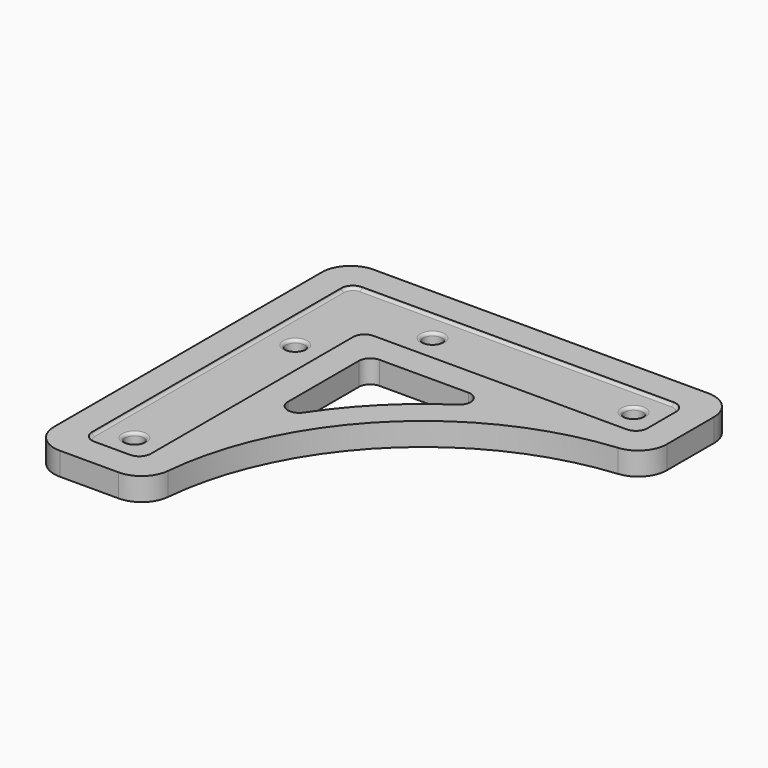
from build123d import *

# Parameters (mm, degrees)
F1_DEPTH = 4
F2_R     = 1.6
F3_DEPTH = 4.001
F4_R     = 5
F5_R     = 1.6
F6_DEPTH = 0.5
F7_R     = 0.49999
F9_DEPTH = 4.001
F10_R    = 2


# Not quite as in the source:
# - a fillet or chamfer is up to 0.001 mm smaller than in the source, because OpenCascade refuses the exact size


with BuildPart() as f1:
    # F0 (on Top) → F1 (new body)
    with BuildSketch(Plane.XY):
        with BuildLine():
            Line((34.1421356237, 14.1421356237), (34.1421356237, 34.1421356237))
            Line((34.1421356237, 34.1421356237), (-34.1421356237, 34.1421356237))
            Line((-34.1421356237, 34.1421356237), (-34.1421356237, -34.1421356237))
            Line((-34.1421356237, -34.1421356237), (-14.1421356237, -34.1421356237))
            ThreePointArc((-14.1421356237, -34.1421356237), (0, 0), (34.1421356237, 14.1421356237))
        make_face()
    extrude(amount=F1_DEPTH)

    # F2 (on face) → F3 (cut, through all)
    with BuildSketch(Plane.XY.offset(4)):
        with Locations((-24.1421356237, -24.1421356237)):
            Circle(F2_R)
        with Locations((-10.8578643763, 24.1421356237)):
            Circle(F2_R)
        with Locations((24.1421356237, 24.1421356237)):
            Circle(F2_R)
        with Locations((-24.1421356237, 10.8578643763)):
            Circle(F2_R)
    extrude(amount=-F3_DEPTH, mode=Mode.SUBTRACT)

    # F4
    f4_edges = [f1.edges().sort_by_distance(p)[0] for p in [
        (-14.142136, -34.142136, 2),
        (-34.142136, -34.142136, 2),
        (34.142136, 14.142136, 2),
        (34.142136, 34.142136, 2),
        (-34.142136, 34.142136, 2),
    ]]
    fillet(f4_edges, radius=F4_R)

    # F5 (on face) → F6 (cut)
    with BuildSketch(Plane.XY.offset(4)):
        with BuildLine():
            ThreePointArc((29.1421356237, 27.1421356237), (28.5563491861, 28.5563491861), (27.1421356237, 29.1421356237))
            Line((27.1421356237, 29.1421356237), (-27.1421356237, 29.1421356237))
            ThreePointArc((-27.1421356237, 29.1421356237), (-28.5563491861, 28.5563491861), (-29.1421356237, 27.1421356237))
            Line((-29.1421356237, 27.1421356237), (-29.1421356237, -27.1421356237))
            ThreePointArc((-29.1421356237, -27.1421356237), (-28.5563491861, -28.5563491861), (-27.1421356237, -29.1421356237))
            Line((-27.1421356237, -29.1421356237), (-20.9070261262, -29.1421356237))
            ThreePointArc((-20.9070261262, -29.1421356237), (-19.4928125639, -28.5563491861), (-18.9070261262, -27.1421356237))
            Line((-18.9070261262, -27.1421356237), (-18.9070261262, 16.9070261262))
            ThreePointArc((-18.9070261262, 16.9070261262), (-18.3212396886, 18.3212396886), (-16.9070261262, 18.9070261262))
            Line((-16.9070261262, 18.9070261262), (27.1421356237, 18.9070261262))
            ThreePointArc((27.1421356237, 18.9070261262), (28.5563491861, 19.4928125639), (29.1421356237, 20.9070261262))
            Line((29.1421356237, 20.9070261262), (29.1421356237, 27.1421356237))
        make_face()
        with Locations((-24.1421356237, -24.1421356237)):
            Circle(F5_R, mode=Mode.SUBTRACT)
        with Locations((-24.1421356237, 10.8578643763)):
            Circle(F5_R, mode=Mode.SUBTRACT)
        with Locations((-10.8578643763, 24.1421356237)):
            Circle(F5_R, mode=Mode.SUBTRACT)
        with Locations((24.1421356237, 24.1421356237)):
            Circle(F5_R, mode=Mode.SUBTRACT)
    extrude(amount=-F6_DEPTH, mode=Mode.SUBTRACT)

    # F7 (radius 0.5 in the source; OpenCascade refuses exactly that, so slightly less here)
    f7_edges = [f1.edges().sort_by_distance(p)[0] for p in [
        (-18.32124, 18.32124, 3.5),
        (5.117555, 18.907026, 3.5),
        (28.556349, 19.492813, 3.5),
        (29.142136, 24.024581, 3.5),
        (28.556349, 28.556349, 3.5),
        (0, 29.142136, 3.5),
        (-28.556349, 28.556349, 3.5),
        (-29.142136, 0, 3.5),
        (-28.556349, -28.556349, 3.5),
        (-24.024581, -29.142136, 3.5),
        (-19.492813, -28.556349, 3.5),
        (-18.907026, -5.117555, 3.5),
        (-25.742136, -24.142136, 3.5),
        (-25.742136, 10.857864, 3.5),
        (-12.457864, 24.142136, 3.5),
        (22.542136, 24.142136, 3.5),
    ]]
    fillet(f7_edges, radius=F7_R)

    # F8 (on face) → F9 (cut, through all)
    with BuildSketch(Plane.XY.offset(4)):
        with BuildLine():
            ThreePointArc((-13.9070261262, -11.1097319823), (-3.5355339059, 3.5355339059), (11.1097319823, 13.9070261262))
            Line((11.1097319823, 13.9070261262), (-13.9070261262, 13.9070261262))
            Line((-13.9070261262, 13.9070261262), (-13.9070261262, -11.1097319823))
        make_face()
    extrude(amount=-F9_DEPTH, mode=Mode.SUBTRACT)

    # F10
    f10_edges = [f1.edges().sort_by_distance(p)[0] for p in [
        (-13.907026, 13.907026, 2),
        (-13.907026, -11.109732, 2),
        (11.109732, 13.907026, 2),
    ]]
    fillet(f10_edges, radius=F10_R)


solid = f1.part
